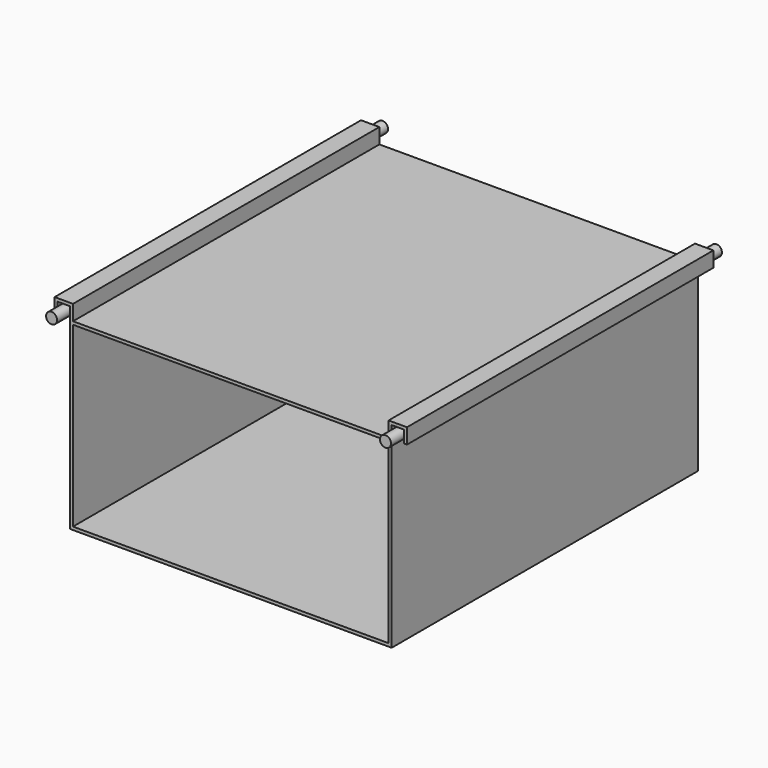
from build123d import *

# Parameters (mm, degrees)
F1_DEPTH = 125
F2_T     = -1
F3_R     = 1.8
F4_DEPTH = 135


# Not quite as in the source:
# - a shell that OpenCascade refuses in one call is made with other operations: the cavity is built on its own and cut out
# - the program builds the solid bodies; features that only make, move or delete a surface that nothing else refers to are left out


with BuildPart() as f1:
    # F0 (on Front) → F1 (new body)
    with BuildSketch(Plane.XZ):
        Polygon((-58.0680891871, 23.6017971635), (-58.0680891871, 19.6017971635), (-57.0680891871, 19.6017971635), (-57.0680891871, 24.6017971635), (-58.0680891871, 24.6017971635), (-63.0680891871, 24.6017971635), (-63.0680891871, 23.6017971635), (-63.0680891871, 19.6017971635), (-62.0680891871, 19.6017971635), (-62.0680891871, 23.6017971635), align=None)
        Polygon((45.9319108129, 19.6017971635), (-5.5680891871, 19.6017971635), (-5.5680891871, -40.3982028365), (46.9319108129, -40.3982028365), (46.9319108129, 19.6017971635), align=None)
        Polygon((45.9319108129, 24.6017971635), (45.9319108129, 19.6017971635), (46.9319108129, 19.6017971635), (46.9319108129, 23.6017971635), (50.9319108129, 23.6017971635), (50.9319108129, 19.6017971635), (51.9319108129, 19.6017971635), (51.9319108129, 23.6017971635), (51.9319108129, 24.6017971635), (46.9319108129, 24.6017971635), align=None)
        Polygon((-57.0680891871, 19.6017971635), (-58.0680891871, 19.6017971635), (-58.0680891871, -10.3982028365), (-58.0680891871, -40.3982028365), (-5.5680891871, -40.3982028365), (-5.5680891871, 19.6017971635), align=None)
    extrude(amount=F1_DEPTH)

    # F2: a shell. OpenCascade refuses it in one call, so the cavity is built on its own and cut out:
    # the body offset inwards by the wall thickness, plus a prism from it out through each open face.
    f2_core = offset(f1.part, amount=F2_T, kind=Kind.INTERSECTION, mode=Mode.PRIVATE)
    f2_exits = [f2_core.faces().sort_by_distance(p)[0] for p in [
        (-5.568089, -124, -10.398203),
        (-5.568089, -1, -10.398203),
    ]]
    add(f2_core, mode=Mode.SUBTRACT)
    extrude(f2_exits, amount=-F2_T, mode=Mode.SUBTRACT)


with BuildPart() as f4:
    # F3 (on Front) → F4 (new body)
    with BuildSketch(Plane.XZ):
        with Locations((48.9230826497, 21.5761251748)):
            Circle(F3_R)
    extrude(amount=F4_DEPTH)


with BuildPart() as f4b:
    # F3 (on Front) → F4, piece 2 (new body)
    with BuildSketch(Plane.XZ):
        with Locations((-60.059261024, 21.5761251748)):
            Circle(F3_R)
    extrude(amount=F4_DEPTH)


with BuildPart() as f4_1:
    # F5: moved
    add(f4.part.moved(Location((0, 5, 0))))


with BuildPart() as f4b_1:
    # F5: moved
    add(f4b.part.moved(Location((0, 5, 0))))


solid = Compound([f1.part, f4_1.part, f4b_1.part])
